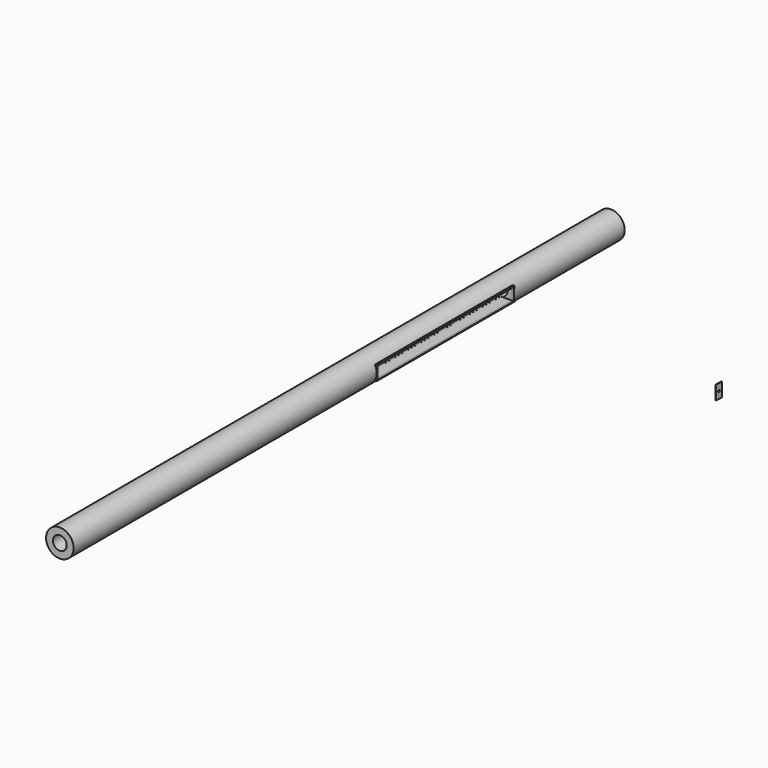
from build123d import *

# Parameters (mm, degrees)
F0_R          = 2
F0_R_2        = 1
F1_DEPTH      = 100
F5_E5_W       = 2.0043330533
F5_E5_H       = 25
F6_DEPTH      = 25
F6_DEPTH_BACK = 1
F9_DEPTH      = 0.3
F10_T         = -0.1
F14_W         = 1.0064751207
F14_H         = 2
F15_DEPTH     = 0.1
F16_D         = 0.3
F17_D         = 0.3


# Not quite as in the source:
# - a feature of the source that left no trace in its solid (it failed there, or was rolled back) is left out


with BuildPart() as f1:
    # F0 (on Front) → F1 (new body)
    with BuildSketch(Plane.XZ):
        Circle(F0_R)
        Circle(F0_R_2, mode=Mode.SUBTRACT)
    extrude(amount=F1_DEPTH)

    # F5_E5 (on explicit) → F6 (cut, two sides)
    with BuildSketch(Plane(origin=(0.9982800111, -45, -1.0022865608), x_dir=(-0.0038684819, 0, 0.9999925174), z_dir=(-0.9999925174, 0, -0.0038684819))) as f6_sk:
        with Locations((1.0021665267, 12.5)):
            Rectangle(F5_E5_W, F5_E5_H)
    extrude(amount=-F6_DEPTH, mode=Mode.SUBTRACT)
    extrude(f6_sk.sketch, amount=F6_DEPTH_BACK, mode=Mode.SUBTRACT)

    # F17 (through all)
    with Locations(Plane(origin=(1.7307944858, 0, 0.0027212049), x_dir=(0, 1, 0), z_dir=(0.9999987641, 0, 0.0015722268))):
        with Locations((-24.1942365289, 0.0004732283)):
            Hole(F17_D / 2)


with BuildPart() as f9:
    # F8 (on face) → F9 (new body)
    with BuildSketch(Plane(origin=(1.7307944858, 0, 0.0027212049), x_dir=(0, 1, 0), z_dir=(0.9999987641, 0, 0.0015722268))):
        Polygon((-45.0004413724, -1.0031352285), (-19.9942365289, -1.0031352285), (-19.9942365289, 0.0004732283), (-24.1942365289, 0.0004732283), (-41.1659032106, 0.0004732283), (-45.0004413724, 0.0004732283), align=None)
        Polygon((-24.1942365289, 0.0004732283), (-19.9942365289, 0.0004732283), (-19.9942365289, 1.0040816851), (-45.0004413724, 1.0040816851), (-45.0004413724, 0.0004732283), (-41.1659032106, 0.0004732283), align=None)
    extrude(amount=F9_DEPTH)

    # F10
    f10_openings = [f9.faces().sort_by_distance(p)[0] for p in [
        (2.030793, -32.497339, 0.003666),
        (1.730794, -32.497339, 0.003194),
    ]]
    offset(amount=F10_T, openings=f10_openings)


with BuildPart() as f15:
    # F14 (on face) → F15 (new body)
    with BuildSketch(Plane(origin=(36.1674841996, -1.8718308958, 0.056863559), x_dir=(0.0516852214, 0.9986634224, 8.1261e-05), z_dir=(0.9986621881, -0.0516852853, 0.0015701254))):
        with Locations((-22.4322800759, -0.0031352285)):
            Rectangle(F14_W, F14_H)
        Polygon((-22.8325207636, -0.9031352285), (-22.8325207636, 0.8968647715), (-22.4346363536, 0.8968647715), (-22.0367519436, 0.8968647715), (-22.0367519436, -0.9031352285), (-22.4346363536, -0.9031352285), align=None, mode=Mode.SUBTRACT)
        Polygon((-22.4346363536, 0.8968647715), (-22.8325207636, 0.8968647715), (-22.8325207636, -0.9031352285), (-22.4346363536, -0.9031352285), (-22.4346363536, -0.0031352285), align=None)
        Polygon((-22.0367519436, 0.8968647715), (-22.4346363536, 0.8968647715), (-22.4346363536, -0.0031352285), (-22.4346363536, -0.9031352285), (-22.0367519436, -0.9031352285), align=None)
    extrude(amount=F15_DEPTH)

    # F16 (through all)
    with Locations(Plane(origin=(36.1674841996, -1.8718308958, 0.056863559), x_dir=(0.0516852214, 0.9986634224, 8.1261e-05), z_dir=(-0.9986621881, 0.0516852853, -0.0015701254))):
        with Locations((-22.4346363536, 0.0031352285)):
            Hole(F16_D / 2)


solid = Compound([f1.part, f9.part, f15.part])
